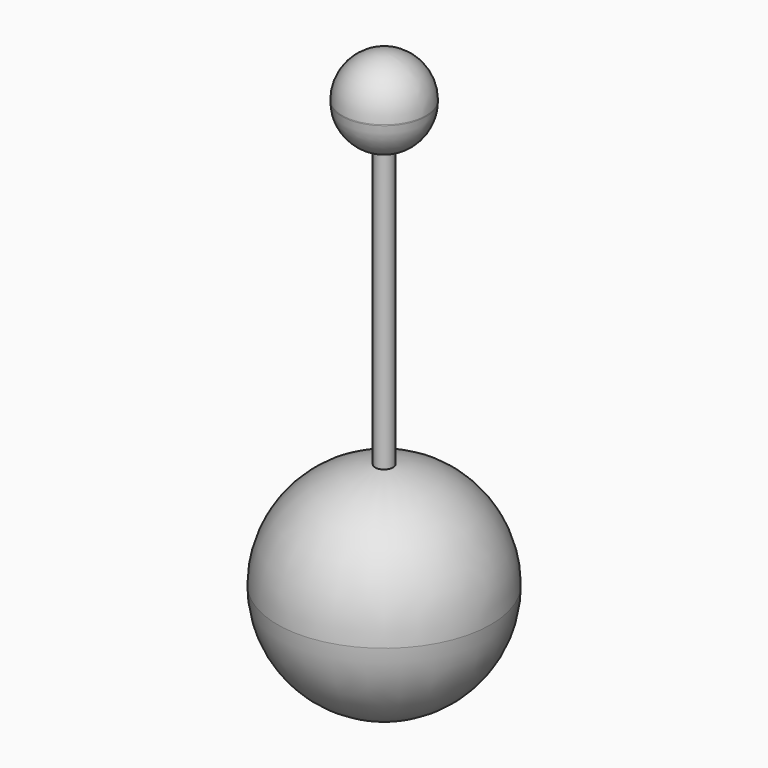
from build123d import *

# Parameters (mm, degrees)
F0_R          = 38.1
F1_DEPTH      = 38.1
F1_DEPTH_BACK = 38.1
F2_R          = 38.09999
F3_R          = 38.09999
F4_R          = 3.175
F5_DEPTH      = 152.4
F6_R          = 15
F7_DEPTH      = 15
F7_DEPTH_BACK = 15
F8_R          = 15


# Not quite as in the source:
# - a fillet or chamfer that OpenCascade refuses, or shapes differently, is made with other operations: its cross-section is extruded or revolved along the edge and cut away or added
# - a fillet or chamfer is up to 0.001 mm smaller than in the source, because OpenCascade refuses the exact size
# - the program builds the solid bodies; features that only make, move or delete a surface that nothing else refers to are left out


with BuildPart() as f1:
    # F0 (on Top) → F1 (new body, two sides)
    with BuildSketch(Plane.XY) as f1_sk:
        Circle(F0_R)
    extrude(amount=F1_DEPTH)
    extrude(f1_sk.sketch, amount=-F1_DEPTH_BACK)

    # F2 (radius 38.1 in the source; OpenCascade refuses exactly that, so slightly less here)
    f2_edges = [f1.edges().sort_by_distance(p)[0] for p in [
        (-38.1, 0, 38.1),
    ]]
    fillet(f2_edges, radius=F2_R)

    # F3 (radius 38.1 in the source; OpenCascade refuses exactly that, so slightly less here)
    f3_edges = [f1.edges().sort_by_distance(p)[0] for p in [
        (-38.1, 0, -38.1),
    ]]
    fillet(f3_edges, radius=F3_R)

    # F4 (on Top) → F5 (join)
    with BuildSketch(Plane.XY):
        Circle(F4_R)
    extrude(amount=F5_DEPTH)

    # F6 (on face) → F7 (join, two sides)
    with BuildSketch(Plane.XY.offset(152.4)) as f7_sk:
        Circle(F6_R)
    extrude(amount=F7_DEPTH)
    extrude(f7_sk.sketch, amount=-F7_DEPTH_BACK)

    # F8
    f8_edges = [f1.edges().sort_by_distance(p)[0] for p in [
        (-15, 0, 167.4),
    ]]
    fillet(f8_edges, radius=F8_R)

    # F9: fillet of radius 14.999 on 1 edges, made by hand

    # F9_s1 → F9_t2 (revolve, cut)
    with BuildSketch(Plane.XZ):
        with BuildLine():
            ThreePointArc((15, 152.0593221194), (11.6752628675, 142.6422319372), (3.175, 137.4))
            Line((3.175, 137.4), (15, 137.4))
            Line((15, 137.4), (15, 152.0593221194))
        make_face()
    revolve(axis=Axis((0, 0, 137.4), (0, 0, 1)), mode=Mode.SUBTRACT)


solid = f1.part
